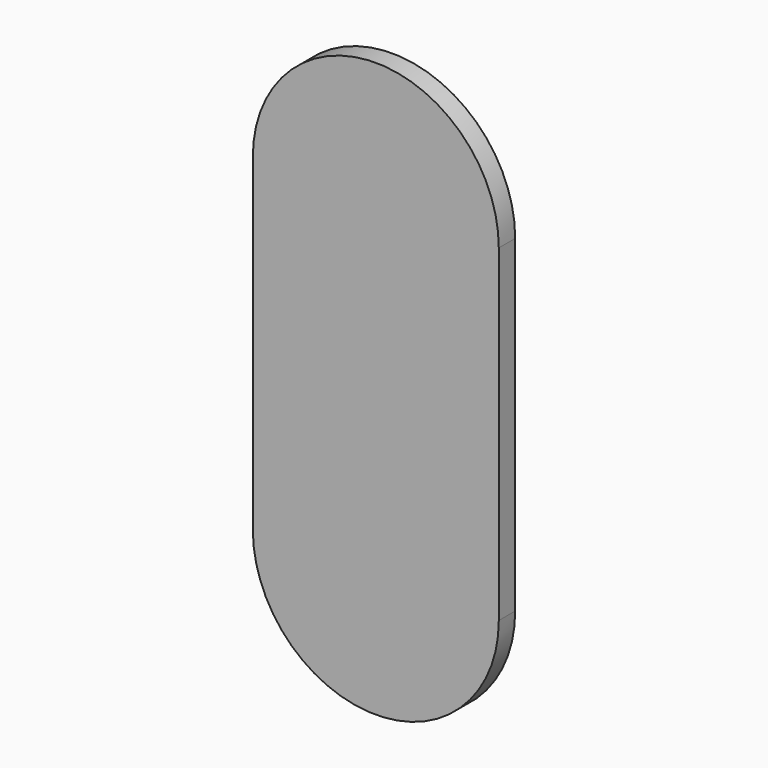
from build123d import *

# Parameters (mm, degrees)
F1_DEPTH = 10


# Not quite as in the source:
# - a feature of the source that left no trace in its solid (it failed there, or was rolled back) is left out


with BuildPart() as f1:
    # F0 (on Front) → F1 (new body)
    with BuildSketch(Plane.XZ):
        with BuildLine():
            ThreePointArc((-60, -80), (0, -140), (60, -80))
            Line((60, -80), (60, 80))
            ThreePointArc((60, 80), (0, 140), (-60, 80))
            Line((-60, 80), (-60, -80))
        make_face()
    extrude(amount=F1_DEPTH)


solid = f1.part
